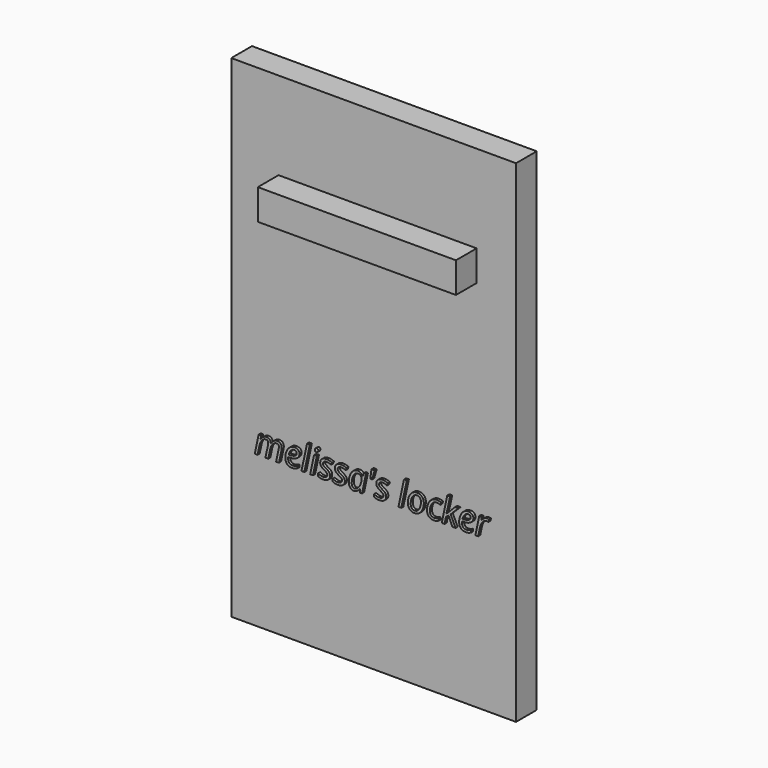
from build123d import *

# Parameters (mm, degrees)
F0_W         = 279.4
F0_H         = 482.6
F1_DEPTH     = 25.4
F4_TEXT_SIZE = 33.577849778
F5_DEPTH     = 2.54
F3_W         = 194.3754330277
F3_H         = 29.9783051014
F6_DEPTH     = 25.4


# Not quite as in the source:
# - the program builds the solid bodies; features that only make, move or delete a surface that nothing else refers to are left out
# - Text() gives the source's letters only with a copy of the font that has no kerning and outlines rounded to 1/6400 em; it was checked with that copy


with BuildPart() as f1:
    # F0 (on Front) → F1 (new body)
    with BuildSketch(Plane.XZ):
        with Locations((-4.5807231218, 77.4175979759)):
            Rectangle(F0_W, F0_H)
    extrude(amount=F1_DEPTH)

    # F4 (on face) → F5 (join)
    with BuildSketch(Plane.XZ.offset(25.4)):
        with Locations((-120.142236352, -13.9678698033)):
            Text("melissa's locker", F4_TEXT_SIZE, font='Open Sans', font_style=FontStyle.ITALIC, text_align=(TextAlign.LEFT, TextAlign.BOTTOM))
    extrude(amount=F5_DEPTH)

    # F3 (on face) → F6 (join)
    with BuildSketch(Plane.XZ.offset(25.4)):
        with Locations((-0.7125549018, 217.6386862993)):
            Rectangle(F3_W, F3_H)
    extrude(amount=F6_DEPTH)


solid = f1.part
